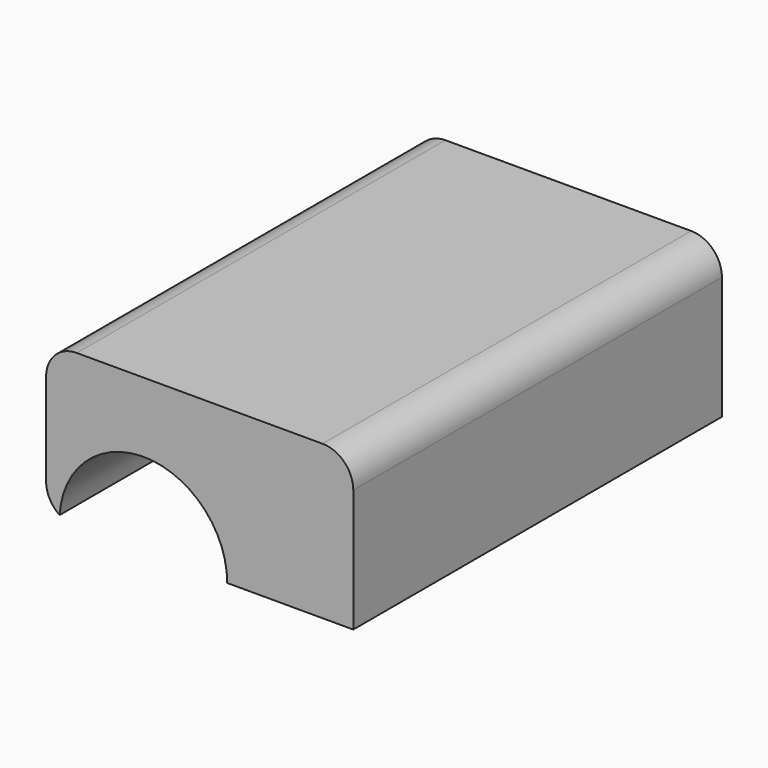
from build123d import *

# Parameters (mm, degrees)
F1_E0_TOP_W = 50.8
F1_E0_TOP_H = 25.4
F2_DEPTH    = 76.2
F3_R        = 5.08
F4_R        = 13.875567501
F5_DEPTH    = 25.4


with BuildPart() as f2:
    # F1_E0_top (on explicit) → F2 (new body)
    with BuildSketch(Plane(origin=(-50.8, 0, 0), x_dir=(1, 0, 0), z_dir=(0, -1, 0))):
        with Locations((25.4, 12.7)):
            Rectangle(F1_E0_TOP_W, F1_E0_TOP_H)
    extrude(amount=F2_DEPTH)

    # F3
    f3_edges = [f2.edges().sort_by_distance(p)[0] for p in [
        (-50.8, -38.1, 0),
        (-50.8, -38.1, 25.4),
        (0, -38.1, 25.4),
    ]]
    fillet(f3_edges, radius=F3_R)

    # F4 (on face) → F5 (cut)
    with BuildSketch(Plane.XZ.offset(76.2)):
        with Locations((-34.7172878683, 0)):
            Circle(F4_R)
    extrude(amount=-F5_DEPTH, mode=Mode.SUBTRACT)


solid = f2.part
